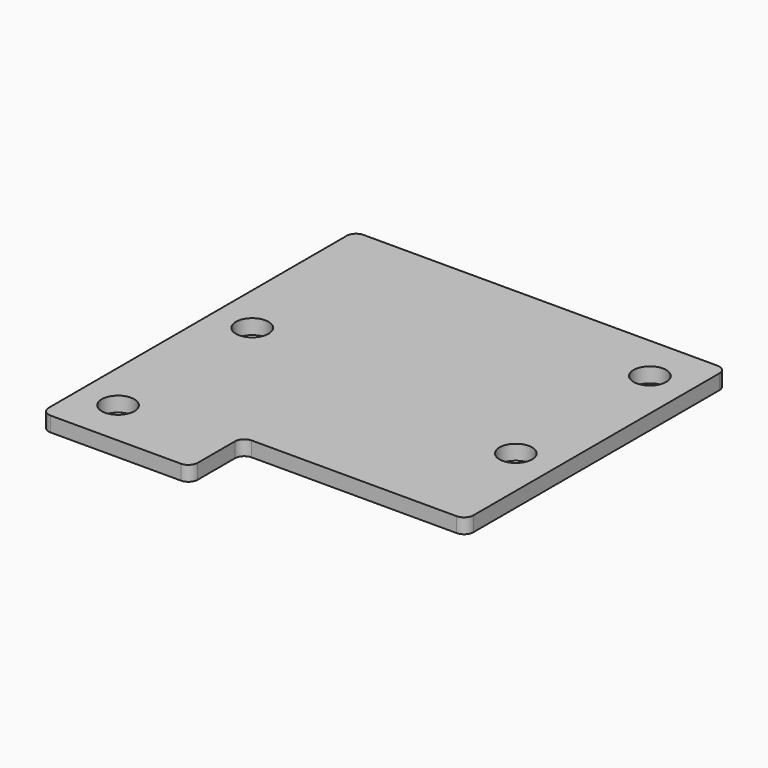
from build123d import *

# Parameters (mm, degrees)
F0_R     = 1.75
F1_DEPTH = 1.6
F2_R     = 1


with BuildPart() as f1:
    # F0 (on Top) → F1 (new body)
    with BuildSketch(Plane.XY):
        Polygon((20, 21), (-20, 21), (-20, -21), (-4, -21), (-4, -14), (20, -14), align=None)
        with Locations((-15.75, -16)):
            Circle(F0_R, mode=Mode.SUBTRACT)
        with Locations((15.75, -2)):
            Circle(F0_R, mode=Mode.SUBTRACT)
        with Locations((-15.75, 2)):
            Circle(F0_R, mode=Mode.SUBTRACT)
        with Locations((15.75, 16)):
            Circle(F0_R, mode=Mode.SUBTRACT)
    extrude(amount=F1_DEPTH)

    # F2
    f2_edges = [f1.edges().sort_by_distance(p)[0] for p in [
        (-20, -21, 0.8),
        (20, 21, 0.8),
        (-20, 21, 0.8),
        (-4, -14, 0.8),
        (-4, -21, 0.8),
        (20, -14, 0.8),
    ]]
    fillet(f2_edges, radius=F2_R)


solid = f1.part
